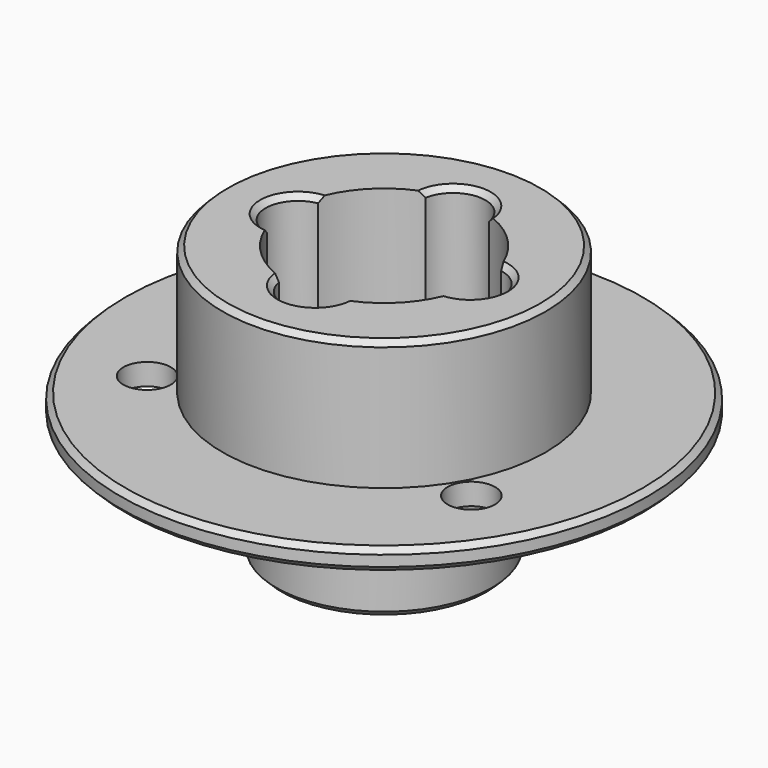
from build123d import *

# Parameters (mm, degrees)
F0_R      = 24.5
F0_R_2    = 15
F1_DEPTH  = 2
F2_R      = 15
F3_DEPTH  = 14
F5_DEPTH  = 11.2
F6_R      = 10
F6_R_2    = 9
F7_DEPTH  = 14
F8_DEPTH  = 25
F10_D     = 4.4
F11_SIZE2 = 0.49999
F11_SIZE  = 0.49999


# Not quite as in the source:
# - a fillet or chamfer is up to 0.001 mm smaller than in the source, because OpenCascade refuses the exact size


with BuildPart() as f1:
    # F0 (on Top) → F1 (new body)
    with BuildSketch(Plane.XY):
        Circle(F0_R)
        Circle(F0_R_2, mode=Mode.SUBTRACT)
    extrude(amount=F1_DEPTH)

    # F2 (on Top) → F3 (join)
    with BuildSketch(Plane.XY):
        Circle(F2_R)
    extrude(amount=F3_DEPTH)

    # F4 (on face) → F5 (cut)
    with BuildSketch(Plane.XY.offset(14)):
        with BuildLine():
            ThreePointArc((7.4375, -2.9467938085), (7.8581168228, -1.5), (8, 0))
            ThreePointArc((8, 0), (7.8581168228, 1.5), (7.4375, 2.9467938085))
            ThreePointArc((7.4375, 2.9467938085), (5.6568542495, 5.6568542495), (2.9467938085, 7.4375))
            ThreePointArc((2.9467938085, 7.4375), (0, 8), (-2.9467938085, 7.4375))
            ThreePointArc((-2.9467938085, 7.4375), (-5.6568542495, 5.6568542495), (-7.4375, 2.9467938085))
            ThreePointArc((-7.4375, 2.9467938085), (-8, 0), (-7.4375, -2.9467938085))
            ThreePointArc((-7.4375, -2.9467938085), (-5.6568542495, -5.6568542495), (-2.9467938085, -7.4375))
            ThreePointArc((-2.9467938085, -7.4375), (0, -8), (2.9467938085, -7.4375))
            ThreePointArc((2.9467938085, -7.4375), (5.6568542495, -5.6568542495), (7.4375, -2.9467938085))
        make_face()
        with BuildLine():
            ThreePointArc((7.4375, 2.9467938085), (7.8581168228, 1.5), (8, 0))
            ThreePointArc((8, 0), (7.8581168228, -1.5), (7.4375, -2.9467938085))
            ThreePointArc((7.4375, -2.9467938085), (11, 0), (7.4375, 2.9467938085))
        make_face()
        with BuildLine():
            ThreePointArc((-2.9467938085, 7.4375), (0, 8), (2.9467938085, 7.4375))
            ThreePointArc((2.9467938085, 7.4375), (0, 11), (-2.9467938085, 7.4375))
        make_face()
        with BuildLine():
            ThreePointArc((-2.9467938085, -7.4375), (0, -11), (2.9467938085, -7.4375))
            ThreePointArc((2.9467938085, -7.4375), (0, -8), (-2.9467938085, -7.4375))
        make_face()
        with BuildLine():
            ThreePointArc((-7.4375, -2.9467938085), (-8, 0), (-7.4375, 2.9467938085))
            ThreePointArc((-7.4375, 2.9467938085), (-11, 0), (-7.4375, -2.9467938085))
        make_face()
    extrude(amount=-F5_DEPTH, mode=Mode.SUBTRACT)

    # F6 (on face) → F7 (join)
    with BuildSketch(Plane.XY.offset(2.8)):
        Circle(F6_R)
        Circle(F6_R_2, mode=Mode.SUBTRACT)
    extrude(amount=-F7_DEPTH)

    # F8 (cut): a face of the model
    f8_faces = [f1.faces().sort_by_distance(p)[0] for p in [
        (0, 0, 0),
    ]]
    extrude(f8_faces, amount=-F8_DEPTH, mode=Mode.SUBTRACT)

    # F10 (through all)
    with Locations(Plane.XY.offset(2)):
        with Locations((0, 17.375), (-15.0471913908, -8.6875), (15.0471913908, -8.6875)):
            Hole(F10_D / 2)

    # F11 (size 0.5 and 0.5 in the source; OpenCascade refuses exactly that, so slightly less here)
    f11_edges = [f1.edges().sort_by_distance(p)[0] for p in [
        (-15, 0, 14),
        (-24.5, 0, 2),
        (-24.5, 0, 0),
        (0, 11, 14),
        (11, 0, 14),
        (0, -11, 14),
        (-11, 0, 14),
        (-10, 0, -11.2),
        (-9, 0, -11.2),
    ]]
    chamfer(f11_edges, length=F11_SIZE, length2=F11_SIZE2)


solid = f1.part
